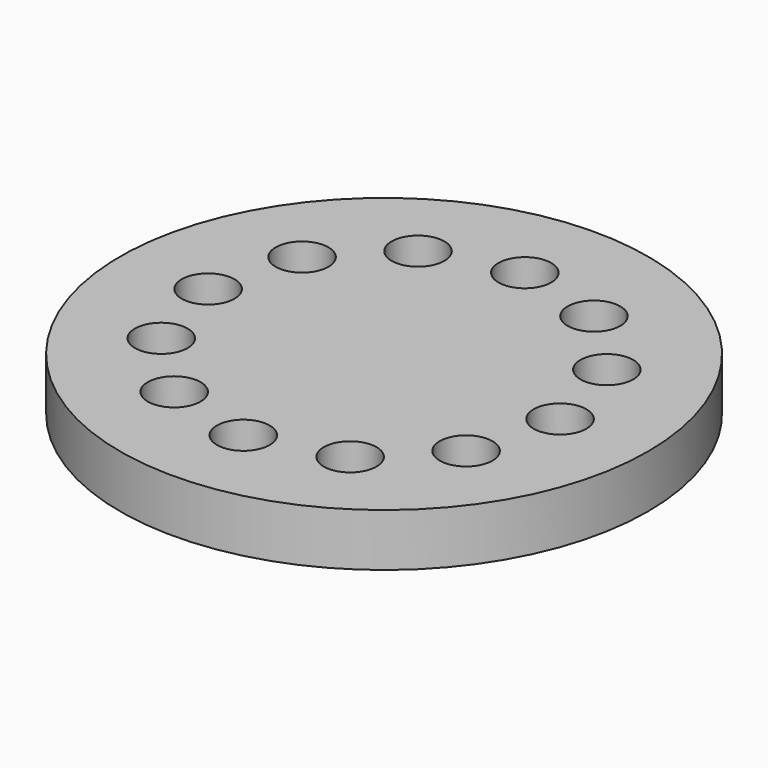
from build123d import *

# Parameters (mm, degrees)
F2_R            = 120
F3_DEPTH        = 24
F4_R            = 12
F5_DEPTH        = 24.001
F5_COPIES_COUNT = 12


# Not quite as in the source:
# - a pattern or mirror of a feature is missing from the dataset's text; its kind, count and spacing are read off the source's solid


with BuildPart() as f3:
    # F2 (on Top) → F3 (new body)
    with BuildSketch(Plane.XY):
        Circle(F2_R)
    extrude(amount=F3_DEPTH)

    # F4 (on face) → F5 (cut, through all)
    with BuildSketch(Plane.XY.offset(24)):
        with Locations((0, 80)):
            Circle(F4_R)
    f5 = extrude(amount=-F5_DEPTH, mode=Mode.SUBTRACT)

    # F5_copies: F5 ×12 about axis
    f5_copies_axis = Axis((0, 0, 0), (0, 0, 1))
    for i in range(1, F5_COPIES_COUNT):
        add(f5.rotate(f5_copies_axis, i * 360 / F5_COPIES_COUNT), mode=Mode.SUBTRACT)


solid = f3.part
